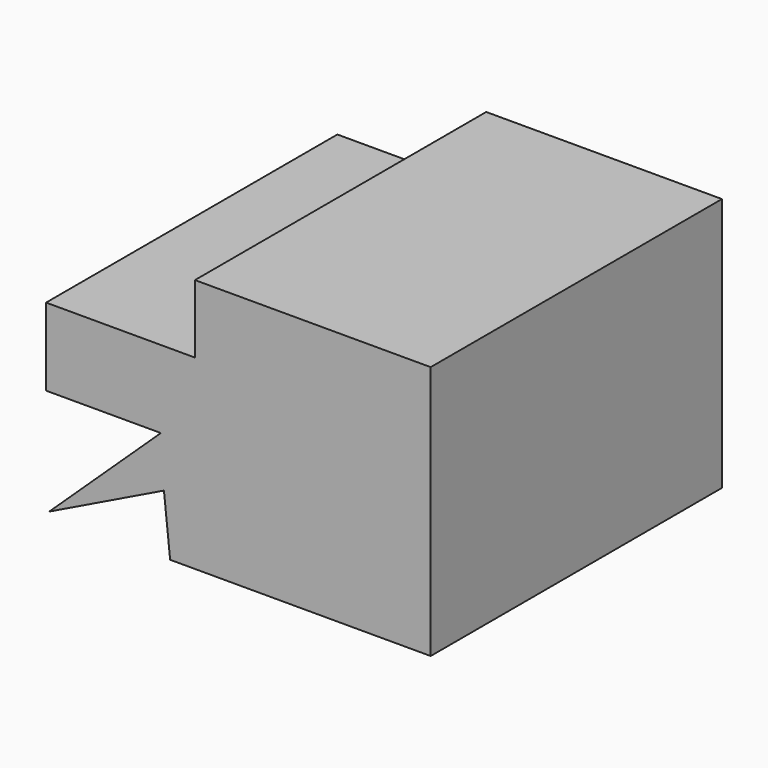
from build123d import *

# Parameters (mm, degrees)
F2_DEPTH = 38.1


# Not quite as in the source:
# - a feature of the source that left no trace in its solid (it failed there, or was rolled back) is left out


with BuildPart() as f2:
    # F1 (on Front) → F2 (new body)
    with BuildSketch(Plane.XZ):
        Polygon((-13.6325350031, 14.11941275), (-12.983366847, 7.9523129389), (14.2817031592, 7.9523129389), (14.2817031592, 34.5682166517), (-10.3866942227, 34.5682166517), (-10.3866942227, 27.4273641407), (-25.9667336941, 27.4273641407), (-25.9667336941, 19.3127579987), (-13.9571195468, 19.3127579987), (-25.642151013, 8.2768965513), align=None)
    extrude(amount=F2_DEPTH)


solid = f2.part
